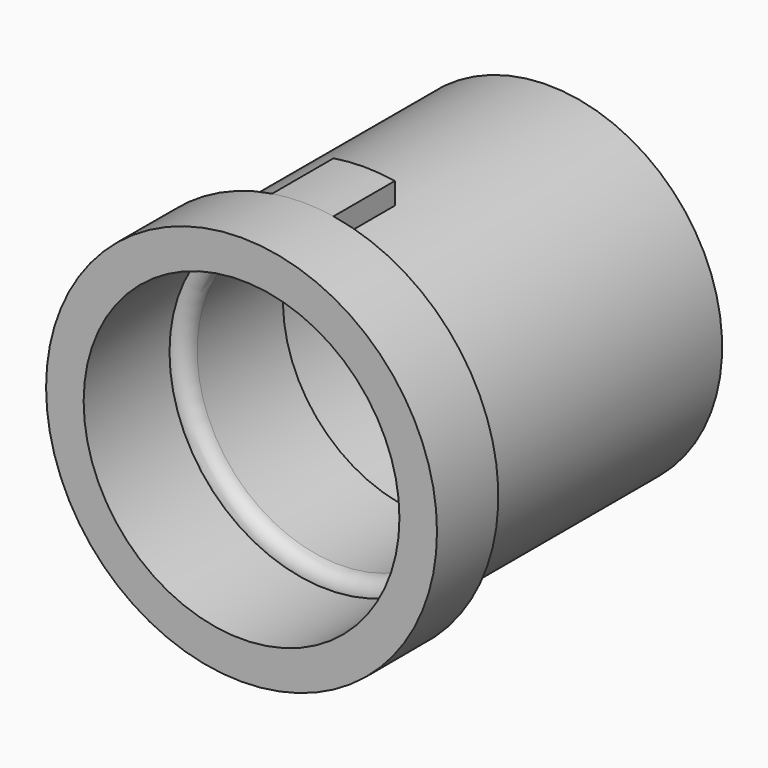
from build123d import *

# Parameters (mm, degrees)
F0_R         = 10.3
F1_DEPTH     = 9
F3_R         = 3.1
F4_DEPTH     = 9.001
F6_DEPTH     = 1.8
F7_T4_ANGLE  = 359.64
F7_S5_R      = 3.1
F7_T6_DEPTH  = 5
F7_T10_ANGLE = 359.64
F7_S11_R     = 3.1
F7_T12_DEPTH = 5
F7_T16_ANGLE = 359.64
F7_S17_R     = 3.1
F7_T18_DEPTH = 5
F9_R         = 12.75
F10_DEPTH    = 25
F11_R        = 3.1
F12_DEPTH    = 34.0010001
F13_R        = 12.75
F13_R_2      = 11.35
F14_DEPTH    = 20
F16_DEPTH    = 5
F17_R        = 10.3
F18_DEPTH    = 34.0010001
F20_START    = -5
F20_DEPTH    = 5
F21_R        = 10.3
F21_R_2      = 9.3
F22_DEPTH    = 8
F23_R        = 0.99999


# Not quite as in the source:
# - a fillet or chamfer that OpenCascade refuses, or shapes differently, is made with other operations: its cross-section is extruded or revolved along the edge and cut away or added
# - a fillet or chamfer is up to 0.001 mm smaller than in the source, because OpenCascade refuses the exact size


with BuildPart() as f1:
    # F0 (on Front) → F1 (new body)
    with BuildSketch(Plane.XZ):
        Circle(F0_R)
    extrude(amount=F1_DEPTH)

    # F3 (on face) → F4 (cut, through all)
    with BuildSketch(Plane.XZ.offset(9)):
        Circle(F3_R)
    extrude(amount=-F4_DEPTH, mode=Mode.SUBTRACT)

    # F5 (on face) → F6 (cut)
    with BuildSketch(Plane.XZ.offset(9)):
        with BuildLine():
            ThreePointArc((-3.0819681678, 0.333874546), (-2.6846787517, 1.55), (-1.8301279224, 2.502125454))
            ThreePointArc((-1.8301279224, 2.502125454), (-6.4951905284, 3.75), (-3.0819681678, 0.333874546))
        make_face()
        with BuildLine():
            ThreePointArc((6.8301270189, 2.5), (4.331189746, 4.9999997741), (1.8301279224, 2.502125454))
            ThreePointArc((1.8301279224, 2.502125454), (2.6846787517, 1.55), (3.0819681678, 0.333874546))
            ThreePointArc((3.0819681678, 0.333874546), (5.5810472546, 0.3354680497), (6.8301270189, 2.5))
        make_face()
        with BuildLine():
            ThreePointArc((1.2518402454, -2.836), (0, -3.1), (-1.2518402454, -2.836))
            ThreePointArc((-1.2518402454, -2.836), (-1.2490795384, -7.1655946774), (2.5, -5))
            ThreePointArc((2.5, -5), (2.1655946774, -3.7509204616), (1.2518402454, -2.836))
        make_face()
    extrude(amount=-F6_DEPTH, mode=Mode.SUBTRACT)

    # F7: fillet of radius 1 on 3 edges, made by hand


with BuildPart() as f7_tool2:
    # F7_s3 → F7_t4 (revolve)
    with BuildSketch(Plane(origin=(0.0078111935, 0, 0.0136280797), x_dir=(0, 1, 0), z_dir=(-0.497276838, 0, -0.8675919239))):
        with BuildLine():
            ThreePointArc((-8.2, -2.499975326), (-7.4928932188, -2.7928685448), (-7.2, -3.499975326))
            Line((-7.2, -3.499975326), (-7.18, -3.499975326))
            Line((-7.18, -3.499975326), (-7.18, -2.479975326))
            Line((-7.18, -2.479975326), (-8.2, -2.479975326))
            Line((-8.2, -2.479975326), (-8.2, -2.499975326))
        make_face()
    revolve(axis=Axis((-4.3301270189, -7.2, 2.5), (0, -1, 0)), revolution_arc=F7_T4_ANGLE)

    # F7_s5 → F7_t6 (cut, symmetric)
    with BuildSketch(Plane.XZ.offset(7.7)):
        Circle(F7_S5_R)
    extrude(amount=F7_T6_DEPTH, both=True, mode=Mode.SUBTRACT)


with BuildPart() as f1_1:
    add(f1.part)

    # F7_t1: union F7_tool2
    add(f7_tool2.part)


with BuildPart() as f7_tool8:
    # F7_s9 → F7_t10 (revolve)
    with BuildSketch(Plane(origin=(0.0078966665, 0, -0.0135787318), x_dir=(0, 1, 0), z_dir=(-0.5027182272, 0, 0.8644503364))):
        with BuildLine():
            ThreePointArc((-8.2, -2.499975326), (-7.4928932188, -2.7928685448), (-7.2, -3.499975326))
            Line((-7.2, -3.499975326), (-7.18, -3.499975326))
            Line((-7.18, -3.499975326), (-7.18, -2.479975326))
            Line((-7.18, -2.479975326), (-8.2, -2.479975326))
            Line((-8.2, -2.479975326), (-8.2, -2.499975326))
        make_face()
    revolve(axis=Axis((4.3301270189, -7.2, 2.5), (0, -1, 0)), revolution_arc=F7_T10_ANGLE)

    # F7_s11 → F7_t12 (cut, symmetric)
    with BuildSketch(Plane.XZ.offset(7.7)):
        Circle(F7_S11_R)
    extrude(amount=F7_T12_DEPTH, both=True, mode=Mode.SUBTRACT)


with BuildPart() as f1_2:
    add(f1_1.part)

    # F7_t7: union F7_tool8
    add(f7_tool8.part)


with BuildPart() as f7_tool14:
    # F7_s15 → F7_t16 (revolve)
    with BuildSketch(Plane(origin=(-0.0157078599, 0, -4.93479e-05), x_dir=(0, 1, 0), z_dir=(0.9999950652, 0, 0.0031415875))):
        with BuildLine():
            ThreePointArc((-8.2, -2.499975326), (-7.4928932188, -2.7928685448), (-7.2, -3.499975326))
            Line((-7.2, -3.499975326), (-7.18, -3.499975326))
            Line((-7.18, -3.499975326), (-7.18, -2.479975326))
            Line((-7.18, -2.479975326), (-8.2, -2.479975326))
            Line((-8.2, -2.479975326), (-8.2, -2.499975326))
        make_face()
    revolve(axis=Axis((0, -7.2, -5), (0, -1, 0)), revolution_arc=F7_T16_ANGLE)

    # F7_s17 → F7_t18 (cut, symmetric)
    with BuildSketch(Plane.XZ.offset(7.7)):
        Circle(F7_S17_R)
    extrude(amount=F7_T18_DEPTH, both=True, mode=Mode.SUBTRACT)


with BuildPart() as f1_3:
    add(f1_2.part)

    # F7_t13: union F7_tool14
    add(f7_tool14.part)

    # F9 (on offset) → F10 (join)
    with BuildSketch(Plane(origin=(0, 0, 0), x_dir=(-1, 0, 0), z_dir=(0, 1, 0))):
        Circle(F9_R)
    extrude(amount=F10_DEPTH)

    # F11 (on face) → F12 (cut, through all)
    with BuildSketch(Plane(origin=(0, 25, 0), x_dir=(-1, 0, 0), z_dir=(0, 1, 0))):
        Circle(F11_R)
    extrude(amount=-F12_DEPTH, mode=Mode.SUBTRACT)

    # F13 (on face) → F14 (cut)
    with BuildSketch(Plane(origin=(0, 25, 0), x_dir=(-1, 0, 0), z_dir=(0, 1, 0))):
        Circle(F13_R)
        Circle(F13_R_2, mode=Mode.SUBTRACT)
    extrude(amount=-F14_DEPTH, mode=Mode.SUBTRACT)

    # F15 (on face) → F16 (join)
    with BuildSketch(Plane(origin=(0, 5, 0), x_dir=(-1, 0, 0), z_dir=(0, 1, 0))):
        with BuildLine():
            ThreePointArc((2, 12.5921602595), (0, 12.75), (-2, 12.5921602595))
            Line((-2, 12.5921602595), (-2, 11.1723990262))
            ThreePointArc((-2, 11.1723990262), (0, 11.35), (2, 11.1723990262))
            Line((2, 11.1723990262), (2, 12.5921602595))
        make_face()
        with BuildLine():
            ThreePointArc((2, -11.1723990262), (0, -11.35), (-2, -11.1723990262))
            Line((-2, -11.1723990262), (-2, -12.5921602595))
            ThreePointArc((-2, -12.5921602595), (0, -12.75), (2, -12.5921602595))
            Line((2, -12.5921602595), (2, -11.1723990262))
        make_face()
    extrude(amount=F16_DEPTH)

    # F17 (on face) → F18 (cut, through all)
    with BuildSketch(Plane.XZ.offset(9)):
        Circle(F17_R)
    extrude(amount=-F18_DEPTH, mode=Mode.SUBTRACT)

    # F19 (on face) → F20 (join)
    with BuildSketch(Plane(origin=(0, 25, 0), x_dir=(-1, 0, 0), z_dir=(0, 1, 0)).offset(F20_START)):
        with BuildLine():
            Line((-7.5, 0), (-10.3, 0))
            ThreePointArc((-10.3, 0), (-9.5744451536, -3.7973675092), (-7.5, -7.0597450379))
            Line((-7.5, -7.0597450379), (-7.5, 0))
        make_face()
    extrude(amount=-F20_DEPTH)

    # F21 (on face) → F22 (join)
    with BuildSketch(Plane.XZ.offset(-15)):
        Circle(F21_R)
        Circle(F21_R_2, mode=Mode.SUBTRACT)
    extrude(amount=F22_DEPTH)

    # F23 (radius 1 in the source; OpenCascade refuses exactly that, so slightly less here)
    f23_edges = [f1_3.edges().sort_by_distance(p)[0] for p in [
        (-9.3, 7, 0),
    ]]
    fillet(f23_edges, radius=F23_R)


solid = f1_3.part
